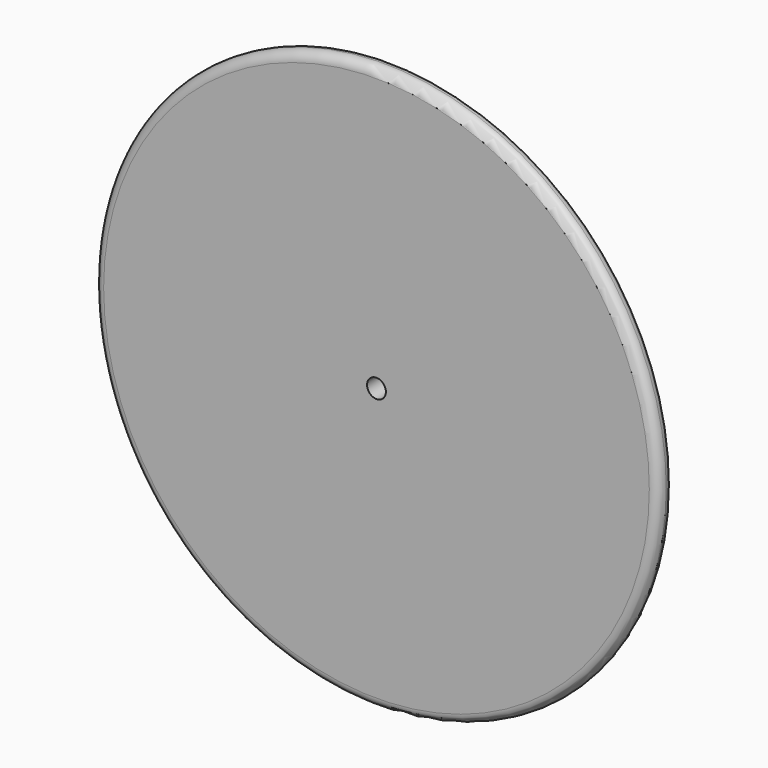
from build123d import *

# Parameters (mm, degrees)
F0_R     = 47.625
F1_DEPTH = 3.175
F2_R     = 1.58749
F3_D     = 3.175


# Not quite as in the source:
# - a fillet or chamfer is up to 0.001 mm smaller than in the source, because OpenCascade refuses the exact size


with BuildPart() as f1:
    # F0 (on Front) → F1 (new body)
    with BuildSketch(Plane.XZ):
        Circle(F0_R)
    extrude(amount=F1_DEPTH)

    # F2 (radius 1.5875 in the source; OpenCascade refuses exactly that, so slightly less here)
    f2_edges = [f1.edges().sort_by_distance(p)[0] for p in [
        (-47.625, -3.175, 0),
        (-47.625, 0, 0),
    ]]
    fillet(f2_edges, radius=F2_R)

    # F3 (through all)
    with Locations(Plane(origin=(0, 0, 0), x_dir=(1, 0, 0), z_dir=(0, 1, 0))):
        with Locations((0, 0)):
            Hole(F3_D / 2)


solid = f1.part
